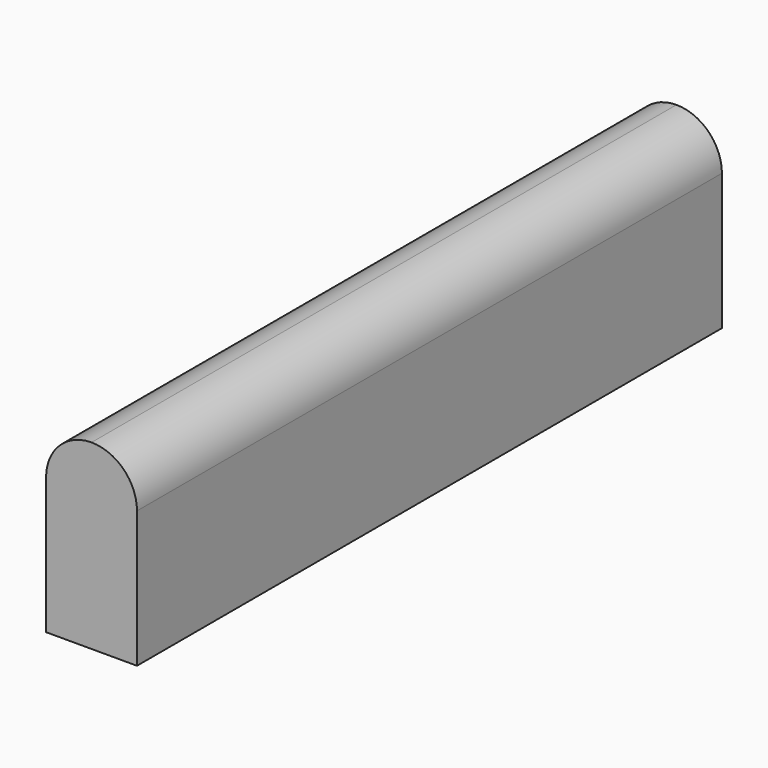
from build123d import *

# Parameters (mm, degrees)
F1_DEPTH = 10
F2_R     = 2.49999
F3_W     = 11.3749653101
F3_H     = 21.1809808388
F4_DEPTH = 25
F5_DEPTH = 25


# Not quite as in the source:
# - a fillet or chamfer is up to 0.001 mm smaller than in the source, because OpenCascade refuses the exact size


with BuildPart() as f1:
    # F0 (on Top) → F1 (new body)
    with BuildSketch(Plane.XY):
        Polygon((-44.6886586582, 25.7738458982), (-44.6886586582, -29.2261541018), (-39.6886586582, -29.2261541018), (-39.6886586582, 20.7738458982), (30.3113413418, 20.7738458982), (30.3113413418, -29.2261541018), (35.3113413418, -29.2261541018), (35.3113413418, 25.7738458982), align=None)
    extrude(amount=F1_DEPTH)

    # F2 (radius 2.5 in the source; OpenCascade refuses exactly that, so slightly less here)
    f2_edges = [f1.edges().sort_by_distance(p)[0] for p in [
        (-44.688659, -1.726154, 10),
        (-39.688659, -4.226154, 10),
        (30.311341, -4.226154, 10),
        (35.311341, -1.726154, 10),
    ]]
    fillet(f2_edges, radius=F2_R)

    # F3 (on Top) → F4 (cut)
    with BuildSketch(Plane.XY):
        Polygon((47.2649559379, 40.0085151196), (-24.1227895021, 40.0085151196), (-24.1227895021, 10.9827276319), (-24.1227895021, -10.1982532069), (-35.4977548122, -10.1982532069), (-35.4977548122, -43.5386821628), (47.2649559379, -43.5386821628), align=None)
        Polygon((-35.4977548122, 10.9827276319), (-35.4977548122, 40.0085151196), (-24.1227895021, 40.0085151196), (-24.1227895021, 54.521407932), (-54.7175332904, 54.521407932), (-54.7175332904, 10.9827276319), align=None)
        with Locations((-29.8102721572, 0.3922372125)):
            Rectangle(F3_W, F3_H)
    extrude(amount=F4_DEPTH, mode=Mode.SUBTRACT)

    # F5 (cut): a face of the model
    f5_faces = [f1.faces().sort_by_distance(p)[0] for p in [
        (-24.1227895021, 23.2738458982, 5),
    ]]
    extrude(f5_faces, amount=-F5_DEPTH, mode=Mode.SUBTRACT)


solid = f1.part
